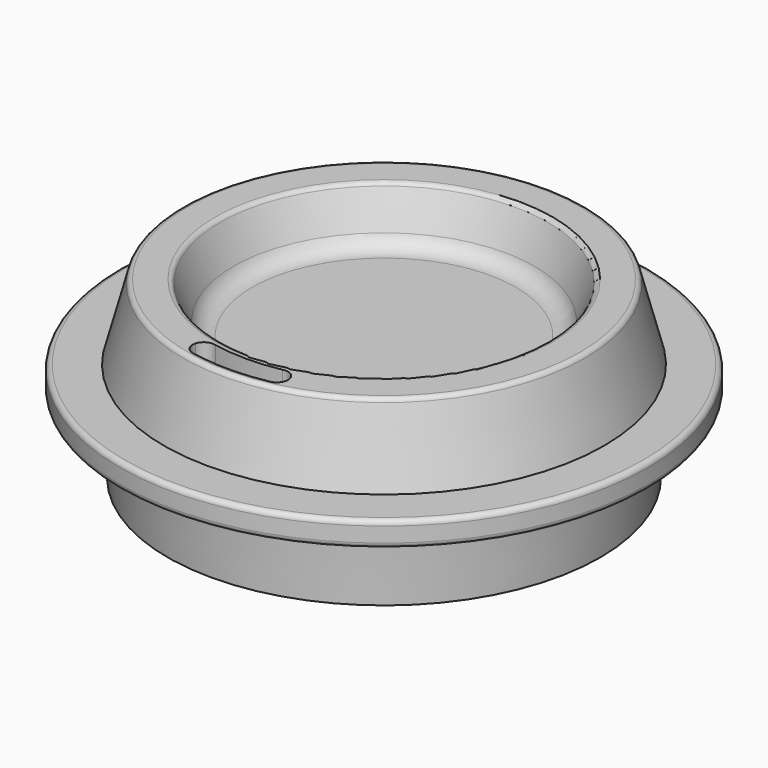
from build123d import *

# Parameters (mm, degrees)
F0_R     = 67.31
F0_R_2   = 56.1246274
F1_DEPTH = 6.35
F0_R_3   = 49.7746274
F2_DEPTH = 19.05
F0_R_4   = 43.4246274
F0_R_5   = 37.0746274
F3_DEPTH = 25.4
F4_SIZE2 = 0.998358
F4_SIZE  = 19.04999
F5_SIZE2 = 19.04999
F5_SIZE  = 5.07999
F6_SIZE2 = 12.7
F6_SIZE  = 5.08
F7_DEPTH = 12.7
F9_DEPTH = 127
F10_R    = 1.27
F11_R    = 5.08


# Not quite as in the source:
# - a fillet or chamfer is up to 0.001 mm smaller than in the source, because OpenCascade refuses the exact size


with BuildPart() as f1:
    # F0 (on Top) → F1 (new body)
    with BuildSketch(Plane.XY):
        Circle(F0_R)
        Circle(F0_R_2, mode=Mode.SUBTRACT)
    extrude(amount=F1_DEPTH)



with BuildPart() as f2:
    # F0 (on Top) → F2 (new body)
    with BuildSketch(Plane.XY):
        Circle(F0_R_2)
        Circle(F0_R_3, mode=Mode.SUBTRACT)
    extrude(amount=-F2_DEPTH)


with BuildPart() as f1_1:
    add(f1.part)

    add(f2.part)  # F3 merges F2
    # F0 (on Top) → F3 (join)
    with BuildSketch(Plane.XY):
        Circle(F0_R_2)
        Circle(F0_R_3, mode=Mode.SUBTRACT)
        Circle(F0_R_3)
        Circle(F0_R_4, mode=Mode.SUBTRACT)
        Circle(F0_R_4)
        Circle(F0_R_5, mode=Mode.SUBTRACT)
    extrude(amount=F3_DEPTH)

    # F4 (size 19.05 and 0.9983681953 in the source; OpenCascade refuses exactly that, so slightly less here)
    f4_edges = [f1_1.edges().sort_by_distance(p)[0] for p in [
        (-56.124627, 0, -19.05),
    ]]
    f4_side = f1_1.faces().sort_by_distance((-56.124627, 0, -9.525))[0]
    chamfer(f4_edges, length=F4_SIZE, length2=F4_SIZE2, reference=f4_side)

    # F5 (size 5.08 and 19.05 in the source; OpenCascade refuses exactly that, so slightly less here)
    f5_edges = [f1_1.edges().sort_by_distance(p)[0] for p in [
        (-56.124627, 0, 25.4),
    ]]
    f5_side = f1_1.faces().sort_by_distance((-54.537183, 0, 25.4))[0]
    chamfer(f5_edges, length=F5_SIZE, length2=F5_SIZE2, reference=f5_side)

    # F6
    f6_edges = [f1_1.edges().sort_by_distance(p)[0] for p in [
        (-37.074627, 0, 25.4),
    ]]
    f6_side = f1_1.faces().sort_by_distance((-49.600877, 0, 25.4))[0]
    chamfer(f6_edges, length=F6_SIZE, length2=F6_SIZE2, reference=f6_side)

    # F0 (on Top) → F7 (join)
    with BuildSketch(Plane.XY):
        Circle(F0_R_5)
    extrude(amount=F7_DEPTH)

    # F8 (on face) → F9 (cut)
    with BuildSketch(Plane.XY.offset(25.4)):
        with BuildLine():
            ThreePointArc((-8.5611625958, -42.9912259739), (-10.7294880172, -43.2766914312), (-12.0608710658, -45.0117836011))
            Line((-12.0608710658, -45.0117836011), (-9.3007380172, -45.7513590225))
            Line((-9.3007380172, -45.7513590225), (-6.5406049686, -46.4909344439))
            ThreePointArc((-6.5406049686, -46.4909344439), (-6.4676843258, -46.1243376168), (-6.4432380172, -45.7513590225))
            ThreePointArc((-6.4432380172, -45.7513590225), (-7.0337308473, -44.0118232391), (-8.5611625958, -42.9912259739))
        make_face()
        with BuildLine():
            ThreePointArc((8.5611625958, -42.9912259739), (0, -43.8353626166), (-8.5611625958, -42.9912259739))
            Line((-8.5611625958, -42.9912259739), (-5.8010295472, -43.7308013952))
            Line((-5.8010295472, -43.7308013952), (-6.5406049686, -46.4909344439))
            Line((-6.5406049686, -46.4909344439), (-7.215923084, -49.0112559618))
            ThreePointArc((-7.215923084, -49.0112559618), (1.2593028677, -49.5235995582), (9.6975364764, -48.581174782))
            ThreePointArc((9.6975364764, -48.581174782), (6.5005137528, -46.3206132005), (8.5611625958, -42.9912259739))
        make_face()
        with BuildLine():
            Line((-9.3007380172, -45.7513590225), (-12.0608710658, -45.0117836011))
            ThreePointArc((-12.0608710658, -45.0117836011), (-11.7754056085, -47.1801090225), (-10.0403134386, -48.5114920711))
            ThreePointArc((-10.0403134386, -48.5114920711), (-9.8689864594, -48.5466359615), (-9.6975364764, -48.581174782))
            ThreePointArc((-9.6975364764, -48.581174782), (-7.7232039405, -48.1339400782), (-6.5406049686, -46.4909344439))
            Line((-6.5406049686, -46.4909344439), (-9.3007380172, -45.7513590225))
        make_face()
        with BuildLine():
            Line((-5.8010295472, -43.7308013952), (-8.5611625958, -42.9912259739))
            ThreePointArc((-8.5611625958, -42.9912259739), (-7.0337308473, -44.0118232391), (-6.4432380172, -45.7513590225))
            ThreePointArc((-6.4432380172, -45.7513590225), (-6.4676843258, -46.1243376168), (-6.5406049686, -46.4909344439))
            Line((-6.5406049686, -46.4909344439), (-5.8010295472, -43.7308013952))
        make_face()
        with BuildLine():
            ThreePointArc((-6.5406049686, -46.4909344439), (-7.7232039405, -48.1339400782), (-9.6975364764, -48.581174782))
            ThreePointArc((-9.6975364764, -48.581174782), (-8.4594634008, -48.8119886491), (-7.215923084, -49.0112559618))
            Line((-7.215923084, -49.0112559618), (-6.5406049686, -46.4909344439))
        make_face()
        with BuildLine():
            ThreePointArc((12.1582380172, -45.7513590225), (11.0402738006, -43.4843518526), (8.5611625958, -42.9912259739))
            ThreePointArc((8.5611625958, -42.9912259739), (6.5005137528, -46.3206132005), (9.6975364764, -48.581174782))
            ThreePointArc((9.6975364764, -48.581174782), (9.8689864594, -48.5466359615), (10.0403134386, -48.5114920711))
            ThreePointArc((10.0403134386, -48.5114920711), (11.5677451871, -47.4908948059), (12.1582380172, -45.7513590225))
        make_face()
    extrude(amount=-F9_DEPTH, mode=Mode.SUBTRACT)

    # F10
    f10_edges = [f1_1.edges().sort_by_distance(p)[0] for p in [
        (-67.31, 0, 6.35),
        (-51.044637, 0, 25.4),
        (-67.31, 0, 0),
        (-42.154627, 0, 25.4),
    ]]
    fillet(f10_edges, radius=F10_R)

    # F11
    f11_edges = [f1_1.edges().sort_by_distance(p)[0] for p in [
        (-37.074627, 0, 12.7),
    ]]
    fillet(f11_edges, radius=F11_R)


solid = f1_1.part
